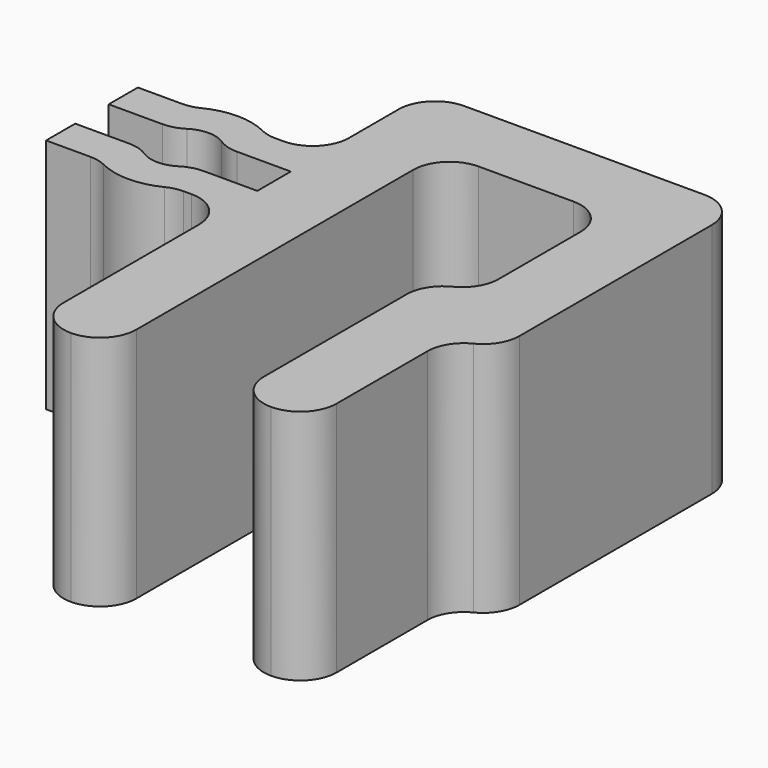
from build123d import *

# Parameters (mm, degrees)
F1_DEPTH = 6.5
F2_R     = 1
F3_R     = 1
F4_R     = 0.99999
F5_R     = 1


# Not quite as in the source:
# - a fillet or chamfer is up to 0.001 mm smaller than in the source, because OpenCascade refuses the exact size


with BuildPart() as f1:
    # F0 (on Top) → F1 (new body)
    with BuildSketch(Plane.XY):
        Polygon((-2.3, 2.3), (2.3, 2.3), (2.3, -2.3), (1.2, -2.3), (1.2, -9.2), (3.2, -9.2), (3.2, -4.3), (4.3, -4.3), (4.3, 4.3), (-4.3, 4.3), (-4.3, 0.6), (-4.3, -0.4), (-4.3, -1.55), (-4.3, -2.3), (-4.3, -2.55), (-4.3, -9.2), (-2.3, -9.2), (-2.3, -2.3), align=None)
        with BuildLine():
            Line((-5.7826505025, -2.55), (-4.3, -2.55))
            Line((-4.3, -2.55), (-4.3, -2.3))
            Line((-4.3, -2.3), (-4.3, -1.55))
            Line((-4.3, -1.55), (-6.1404547021, -1.55))
            ThreePointArc((-6.1404547021, -1.55), (-6.8, -1.85), (-7.4595452979, -1.55))
            Line((-7.4595452979, -1.55), (-9.3, -1.55))
            Line((-9.3, -1.55), (-9.3, -2.55))
            Line((-9.3, -2.55), (-7.8173494975, -2.55))
            Line((-7.8173494975, -2.55), (-5.7826505025, -2.55))
        make_face()
        with BuildLine():
            ThreePointArc((-7.8173494975, -2.55), (-6.8, -2.85), (-5.7826505025, -2.55))
            Line((-5.7826505025, -2.55), (-7.8173494975, -2.55))
        make_face()
        with BuildLine():
            Line((-6.1404547021, -0.4), (-4.3, -0.4))
            Line((-4.3, -0.4), (-4.3, 0.6))
            Line((-4.3, 0.6), (-5.7826505025, 0.6))
            ThreePointArc((-5.7826505025, 0.6), (-6.8, 0.9), (-7.8173494975, 0.6))
            Line((-7.8173494975, 0.6), (-9.3, 0.6))
            Line((-9.3, 0.6), (-9.3, -0.4))
            Line((-9.3, -0.4), (-7.4595452979, -0.4))
            ThreePointArc((-7.4595452979, -0.4), (-6.8, -0.1), (-6.1404547021, -0.4))
        make_face()
    extrude(amount=F1_DEPTH)

    # F2
    f2_edges = [f1.edges().sort_by_distance(p)[0] for p in [
        (-7.817349, -2.55, 3.25),
        (-7.817349, 0.6, 3.25),
        (-5.782651, 0.6, 3.25),
    ]]
    fillet(f2_edges, radius=F2_R)

    # F3
    f3_edges = [f1.edges().sort_by_distance(p)[0] for p in [
        (-6.140455, -1.55, 3.25),
        (-7.459545, -1.55, 3.25),
        (-7.459545, -0.4, 3.25),
        (-6.140455, -0.4, 3.25),
    ]]
    fillet(f3_edges, radius=F3_R)

    # F4 (radius 1 in the source; OpenCascade refuses exactly that, so slightly less here)
    f4_edges = [f1.edges().sort_by_distance(p)[0] for p in [
        (-4.3, -9.2, 3.25),
        (-2.3, -9.2, 3.25),
        (1.2, -9.2, 3.25),
        (3.2, -9.2, 3.25),
        (-4.3, 4.3, 3.25),
        (4.3, -4.3, 3.25),
        (4.3, 4.3, 3.25),
        (1.2, -2.3, 3.25),
    ]]
    fillet(f4_edges, radius=F4_R)

    # F5
    f5_edges = [f1.edges().sort_by_distance(p)[0] for p in [
        (-2.3, 2.3, 3.25),
        (2.3, 2.3, 3.25),
        (2.3, -2.3, 3.25),
        (3.2, -4.3, 3.25),
        (-4.3, 0.6, 3.25),
        (-4.3, -2.55, 3.25),
        (-5.782651, -2.55, 3.25),
    ]]
    fillet(f5_edges, radius=F5_R)


solid = f1.part
